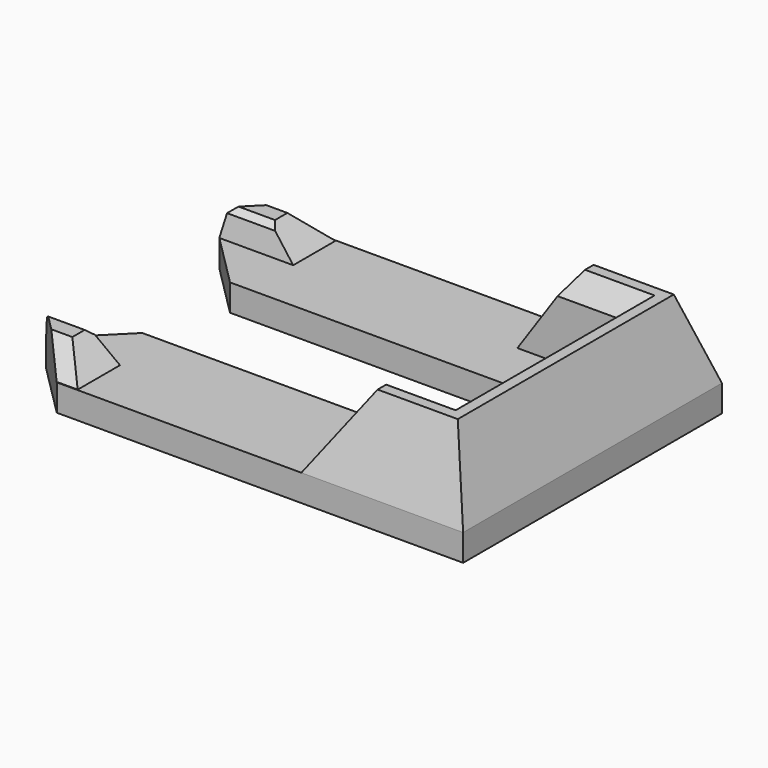
from build123d import *

# Parameters (mm, degrees)
F0_W           = 172
F0_H           = 60.5
F4_DEPTH       = 5
F6_SIZE2       = 4
F6_SIZE        = 3
F9_DEPTH       = 5
F10_SIZE       = 4.99999
F11_SIZE2      = 0.99999
F11_SIZE       = 4.99999
F12_SIZE       = 1
F14_W          = 132
F14_H          = 20.5
F15_DEPTH      = 12.5
F17_DEPTH      = 25
F17_DEPTH_BACK = 25


# Not quite as in the source:
# - a fillet or chamfer is up to 0.001 mm smaller than in the source, because OpenCascade refuses the exact size


with BuildPart() as f4:
    # F0 (on Top) → F4 (new body)
    with BuildSketch(Plane.XY):
        Rectangle(F0_W, F0_H)
    extrude(amount=-F4_DEPTH)

    # F3 (on Top) → F5 section 0
    with BuildSketch(Plane.XY):
        Polygon((-86, 0), (-86, -30.25), (-55.75, -30.25), (-55.75, -20.25), (-76, -20.25), (-76, 0), align=None)
    # F2 (on offset) → F5 section 1
    with BuildSketch(Plane.XY.offset(15)):
        Polygon((-76, -20.25), (-76, 0), (-81, 0), (-81, -25.25), (-66, -25.25), (-66, -20.25), align=None)
    loft()

    # F6
    f6_edges = [f4.edges().sort_by_distance(p)[0] for p in [
        (-76, -10.125, 15),
        (-71, -20.25, 15),
    ]]
    chamfer(f6_edges, length=F6_SIZE, length2=F6_SIZE2)

    # F7: F4 across plane


with BuildPart() as f4_1:
    add(f4.part)
    add(f4.part.mirror(Plane.YZ))

    # F8 (on face) → F9 (join)
    with BuildSketch(Plane.XY):
        Polygon((13.8189587742, -20.25), (0, -20.25), (-13.8189587742, -20.25), (-13.8189587742, -30.1344580948), (0, -30.1344580948), (13.8189587742, -30.1344580948), align=None)
    extrude(amount=F9_DEPTH)

    # F10 (size 5 in the source; OpenCascade refuses exactly that, so slightly less here)
    f10_edges = [f4_1.edges().sort_by_distance(p)[0] for p in [
        (13.818959, -25.192229, 5),
        (0, -30.134458, 5),
        (-13.818959, -25.192229, 5),
    ]]
    chamfer(f10_edges, length=F10_SIZE)

    # F11 (size 5 and 1 in the source; OpenCascade refuses exactly that, so slightly less here)
    f11_edges = [f4_1.edges().sort_by_distance(p)[0] for p in [
        (0, -20.25, 5),
    ]]
    f11_side = f4_1.faces().sort_by_distance((0, -20.25, 2.315943))[0]
    chamfer(f11_edges, length=F11_SIZE, length2=F11_SIZE2, reference=f11_side)

    # F12
    f12_edges = [f4_1.edges().sort_by_distance(p)[0] for p in [
        (0, -21.24999, 5),
    ]]
    chamfer(f12_edges, length=F12_SIZE)

    # F13: F4 across plane


with BuildPart() as f4_2:
    add(f4_1.part)
    add(f4_1.part.mirror(Plane.XZ))

    # F14 (on Top) → F15 (cut, symmetric)
    with BuildSketch(Plane.XY):
        Rectangle(F14_W, F14_H)
    extrude(amount=F15_DEPTH, both=True, mode=Mode.SUBTRACT)


with BuildPart() as f17:
    # F16 (on Top) → F17 (new body, two sides)
    with BuildSketch(Plane.XY) as f17_sk:
        Polygon((23.7979591321, 44.0479591321), (0, 20.25), (18.644013716, 1.605986284), (18.644013716, -1.605986284), (0, -20.25), (26.894013716, -47.144013716), (91.0670285058, -47.144013716), (91.0670285058, 44.0479591321), align=None)
    extrude(amount=F17_DEPTH)
    extrude(f17_sk.sketch, amount=-F17_DEPTH_BACK)

    # F18: intersect F4
    add(f4_2.part, mode=Mode.INTERSECT)


solid = f17.part
